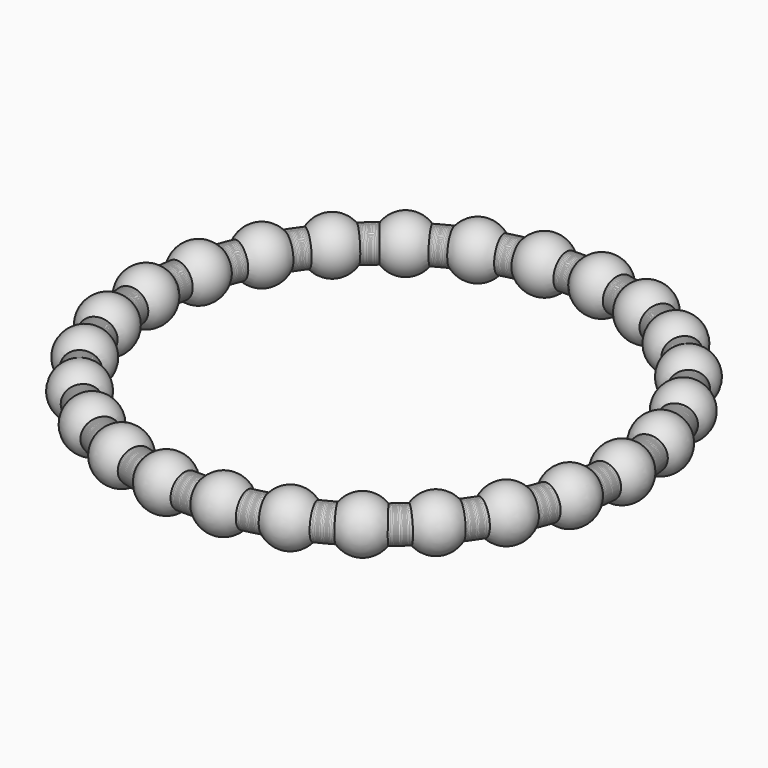
from build123d import *

# Parameters (mm, degrees)
F0_R     = 3.5
F4_COUNT = 26


with BuildPart() as f1:
    # F0 (on Front) → F1 (revolve)
    with BuildSketch(Plane.XZ):
        with Locations((50, 0)):
            Circle(F0_R)
    revolve(axis=Axis((0, 0, 1.4227576994), (0, 0, -1)))

    # F2 (on Front) → F3 (revolve)
    with BuildSketch(Plane.XZ):
        with BuildLine():
            Line((50, 5.5), (50, 3.5))
            ThreePointArc((50, 3.5), (52.4748737342, 2.4748737342), (53.5, 0))
            ThreePointArc((53.5, 0), (52.4748737342, -2.4748737342), (50, -3.5))
            Line((50, -3.5), (50, -5.5))
            ThreePointArc((50, -5.5), (55.5, 0), (50, 5.5))
        make_face()
    revolve(axis=Axis((50, 0, 0), (0, 0, -1)))


with BuildPart() as f4_1:
    # F4: instance of F1
    add(f1.part.rotate(Axis((0, 0, 1.4227576994), (0, 0, -1)), 1 * 360 / F4_COUNT))


with BuildPart() as f4_2:
    # F4: instance of F1
    add(f1.part.rotate(Axis((0, 0, 1.4227576994), (0, 0, -1)), 2 * 360 / F4_COUNT))


with BuildPart() as f4_3:
    # F4: instance of F1
    add(f1.part.rotate(Axis((0, 0, 1.4227576994), (0, 0, -1)), 3 * 360 / F4_COUNT))


with BuildPart() as f4_4:
    # F4: instance of F1
    add(f1.part.rotate(Axis((0, 0, 1.4227576994), (0, 0, -1)), 4 * 360 / F4_COUNT))


with BuildPart() as f4_5:
    # F4: instance of F1
    add(f1.part.rotate(Axis((0, 0, 1.4227576994), (0, 0, -1)), 5 * 360 / F4_COUNT))


with BuildPart() as f4_6:
    # F4: instance of F1
    add(f1.part.rotate(Axis((0, 0, 1.4227576994), (0, 0, -1)), 6 * 360 / F4_COUNT))


with BuildPart() as f4_7:
    # F4: instance of F1
    add(f1.part.rotate(Axis((0, 0, 1.4227576994), (0, 0, -1)), 7 * 360 / F4_COUNT))


with BuildPart() as f4_8:
    # F4: instance of F1
    add(f1.part.rotate(Axis((0, 0, 1.4227576994), (0, 0, -1)), 8 * 360 / F4_COUNT))


with BuildPart() as f4_9:
    # F4: instance of F1
    add(f1.part.rotate(Axis((0, 0, 1.4227576994), (0, 0, -1)), 9 * 360 / F4_COUNT))


with BuildPart() as f4_10:
    # F4: instance of F1
    add(f1.part.rotate(Axis((0, 0, 1.4227576994), (0, 0, -1)), 10 * 360 / F4_COUNT))


with BuildPart() as f4_11:
    # F4: instance of F1
    add(f1.part.rotate(Axis((0, 0, 1.4227576994), (0, 0, -1)), 11 * 360 / F4_COUNT))


with BuildPart() as f4_12:
    # F4: instance of F1
    add(f1.part.rotate(Axis((0, 0, 1.4227576994), (0, 0, -1)), 12 * 360 / F4_COUNT))


with BuildPart() as f4_13:
    # F4: instance of F1
    add(f1.part.rotate(Axis((0, 0, 1.4227576994), (0, 0, -1)), 13 * 360 / F4_COUNT))


with BuildPart() as f4_14:
    # F4: instance of F1
    add(f1.part.rotate(Axis((0, 0, 1.4227576994), (0, 0, -1)), 14 * 360 / F4_COUNT))


with BuildPart() as f4_15:
    # F4: instance of F1
    add(f1.part.rotate(Axis((0, 0, 1.4227576994), (0, 0, -1)), 15 * 360 / F4_COUNT))


with BuildPart() as f4_16:
    # F4: instance of F1
    add(f1.part.rotate(Axis((0, 0, 1.4227576994), (0, 0, -1)), 16 * 360 / F4_COUNT))


with BuildPart() as f4_17:
    # F4: instance of F1
    add(f1.part.rotate(Axis((0, 0, 1.4227576994), (0, 0, -1)), 17 * 360 / F4_COUNT))


with BuildPart() as f4_18:
    # F4: instance of F1
    add(f1.part.rotate(Axis((0, 0, 1.4227576994), (0, 0, -1)), 18 * 360 / F4_COUNT))


with BuildPart() as f4_19:
    # F4: instance of F1
    add(f1.part.rotate(Axis((0, 0, 1.4227576994), (0, 0, -1)), 19 * 360 / F4_COUNT))


with BuildPart() as f4_20:
    # F4: instance of F1
    add(f1.part.rotate(Axis((0, 0, 1.4227576994), (0, 0, -1)), 20 * 360 / F4_COUNT))


with BuildPart() as f4_21:
    # F4: instance of F1
    add(f1.part.rotate(Axis((0, 0, 1.4227576994), (0, 0, -1)), 21 * 360 / F4_COUNT))


with BuildPart() as f4_22:
    # F4: instance of F1
    add(f1.part.rotate(Axis((0, 0, 1.4227576994), (0, 0, -1)), 22 * 360 / F4_COUNT))


with BuildPart() as f4_23:
    # F4: instance of F1
    add(f1.part.rotate(Axis((0, 0, 1.4227576994), (0, 0, -1)), 23 * 360 / F4_COUNT))


with BuildPart() as f4_24:
    # F4: instance of F1
    add(f1.part.rotate(Axis((0, 0, 1.4227576994), (0, 0, -1)), 24 * 360 / F4_COUNT))


with BuildPart() as f4_25:
    # F4: instance of F1
    add(f1.part.rotate(Axis((0, 0, 1.4227576994), (0, 0, -1)), 25 * 360 / F4_COUNT))


solid = Compound([f1.part, f4_1.part, f4_2.part, f4_3.part, f4_4.part, f4_5.part, f4_6.part, f4_7.part, f4_8.part, f4_9.part, f4_10.part, f4_11.part, f4_12.part, f4_13.part, f4_14.part, f4_15.part, f4_16.part, f4_17.part, f4_18.part, f4_19.part, f4_20.part, f4_21.part, f4_22.part, f4_23.part, f4_24.part, f4_25.part])
